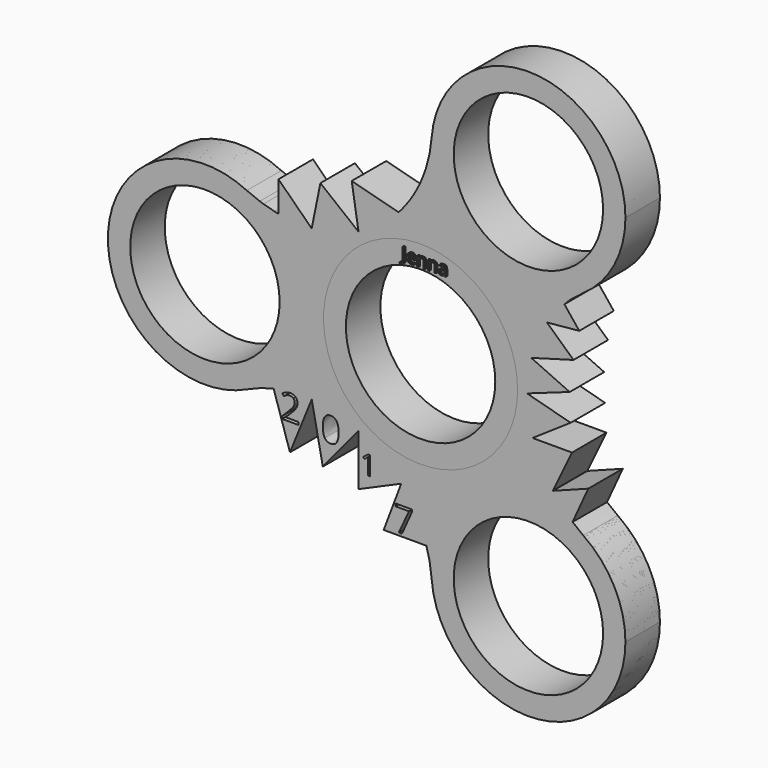
from build123d import *

# Parameters (mm, degrees)
F0_R         = 14.2875
F0_R_2       = 10.9982
F3_DEPTH     = 6.35
F1_R         = 10.9982
F1_R_2       = 14.2875
F2_TEXT_SIZE = 2.6101414632
F4_DEPTH     = 6.604


# Not quite as in the source:
# - Text() gives the source's letters only with a copy of the font that has no kerning and outlines rounded to 1/6400 em; it was checked with that copy


with BuildPart() as f3:
    # F0 (on Front) → F3 (new body)
    with BuildSketch(Plane.XZ):
        with BuildLine():
            ThreePointArc((-25.5840395423, 12.8885060377), (-19.6622207108, 7.6169710585), (-17.4625, 0))
            ThreePointArc((-17.4625, 0), (-19.6622207439, -7.616971111), (-25.5840396543, -12.8885060913))
            ThreePointArc((-25.5840396543, -12.8885060913), (-7.837759128, -13.5753968045), (1.630246118, -28.6006810957))
            ThreePointArc((1.630246118, -28.6006810957), (8.7312501488, -15.1229685276), (23.9537936189, -15.7121752949))
            ThreePointArc((23.9537936189, -15.7121752949), (15.6755180632, -1.024e-07), (23.95379345, 15.7121751791))
            ThreePointArc((23.95379345, 15.7121751791), (8.7312498422, 15.1229687047), (1.630246157, 28.6006815976))
            ThreePointArc((1.630246157, 28.6006815976), (-7.8377588563, 13.5753969614), (-25.5840395423, 12.8885060377))
        make_face()
        Circle(F0_R, mode=Mode.SUBTRACT)
        with BuildLine():
            ThreePointArc((-25.5840396543, -12.8885060913), (-19.6622207439, -7.616971111), (-17.4625, 0))
            ThreePointArc((-17.4625, 0), (-19.6622207108, 7.6169710585), (-25.5840395423, 12.8885060377))
            ThreePointArc((-25.5840395423, 12.8885060377), (-46.0375, 6.21e-08), (-25.5840396543, -12.8885060913))
        make_face()
        with Locations((-31.75, 0)):
            Circle(F0_R_2, mode=Mode.SUBTRACT)
        Circle(F0_R)
        Circle(F0_R_2, mode=Mode.SUBTRACT)
        with BuildLine():
            ThreePointArc((30.1625, 27.4963065702), (16.4276009942, 41.7731160313), (1.630246157, 28.6006815976))
            ThreePointArc((1.630246157, 28.6006815976), (8.7312498422, 15.1229687047), (23.95379345, 15.7121751791))
            ThreePointArc((23.95379345, 15.7121751791), (28.5153800905, 20.8364681775), (30.1625, 27.4963065702))
        make_face()
        with Locations((15.875, 27.4963065702)):
            Circle(F0_R_2, mode=Mode.SUBTRACT)
        with BuildLine():
            ThreePointArc((23.9537936189, -15.7121752949), (8.7312501488, -15.1229685276), (1.630246118, -28.6006810957))
            ThreePointArc((1.630246118, -28.6006810957), (16.4276007427, -41.7731160411), (30.1625, -27.4963065702))
            ThreePointArc((30.1625, -27.4963065702), (28.5153801383, -20.8364682681), (23.9537936189, -15.7121752949))
        make_face()
        with Locations((15.875, -27.4963065702)):
            Circle(F0_R_2, mode=Mode.SUBTRACT)
    extrude(amount=F3_DEPTH)

    # F2 (on face) → F4 (join)
    with BuildSketch(Plane.XZ):
        with Locations((-2.6774271391, 11.3784307614)):
            Text('Jenna', F2_TEXT_SIZE, font='Open Sans', text_align=(TextAlign.LEFT, TextAlign.BOTTOM))
    extrude(amount=F4_DEPTH)


with BuildPart() as f3b:
    # F1 (on face) → F3, piece 2 (new body)
    with BuildSketch(Plane.XZ):
        with BuildLine():
            ThreePointArc((1.6302461293, -28.6006812411), (16.4276008155, -41.7731160383), (30.1625, -27.4963065702))
            ThreePointArc((30.1625, -27.4963065702), (28.5153800921, -20.8364681805), (23.9537934556, -15.7121751829))
            ThreePointArc((23.9537934556, -15.7121751829), (8.73125, -15.1229686136), (1.6302461293, -28.6006812411))
        make_face()
        with Locations((15.875, -27.4963065702)):
            Circle(F1_R, mode=Mode.SUBTRACT)
        with BuildLine():
            ThreePointArc((1.6302461293, -28.6006812411), (8.73125, -15.1229686136), (23.9537934556, -15.7121751829))
            ThreePointArc((23.9537934556, -15.7121751829), (23.1461983486, -15.126858727), (22.3703450113, -14.5000758225))
            ThreePointArc((22.3703450113, -14.5000758225), (20.8277143031, -13.0289504814), (19.4590986494, -11.3946890384))
            ThreePointArc((19.4590986494, -11.3946890384), (17.7185481854, -8.5828594055), (16.4904950244, -5.5123892076))
            ThreePointArc((16.4904950244, -5.5123892076), (15.8803636609, -2.7861542592), (15.6755180632, 0))
            ThreePointArc((15.6755180632, 0), (15.8305224894, 2.4252097364), (16.2930133142, 4.8109529906))
            ThreePointArc((16.2930133142, 4.8109529906), (17.2447328672, 7.5713043086), (18.6071112176, 10.1537904627))
            ThreePointArc((18.6071112176, 10.1537904627), (19.7971807554, 11.8341558729), (21.1616623158, 13.3762594646))
            ThreePointArc((21.1616623158, 13.3762594646), (22.5018016331, 14.6110662389), (23.9537934556, 15.7121751829))
            ThreePointArc((23.9537934556, 15.7121751829), (8.7312498543, 15.1229686977), (1.6302461553, 28.6006815765))
            ThreePointArc((1.6302461553, 28.6006815765), (0.1447682107, 22.5639205285), (-3.2052619846, 17.3268959567))
            ThreePointArc((-3.2052619846, 17.3268959567), (-5.9528221166, 14.818154103), (-9.1356129248, 12.8913134143))
            ThreePointArc((-9.1356129248, 12.8913134143), (-12.4975441494, 11.654923986), (-16.0314960729, 11.069753771))
            ThreePointArc((-16.0314960729, 11.069753771), (-18.4857916979, 11.0563120371), (-20.921446323, 11.3585275925))
            ThreePointArc((-20.921446323, 11.3585275925), (-23.302213479, 11.9727559214), (-25.584039585, 12.8885060581))
            ThreePointArc((-25.584039585, 12.8885060581), (-19.6622207234, 7.6169710785), (-17.4625, 0))
            ThreePointArc((-17.4625, 0), (-19.6622207234, -7.6169710785), (-25.584039585, -12.8885060581))
            ThreePointArc((-25.584039585, -12.8885060581), (-23.6486295526, -12.0901240045), (-21.6372972258, -11.508945746))
            ThreePointArc((-21.6372972258, -11.508945746), (-18.8452797946, -11.08095523), (-16.0206686307, -11.0705153746))
            ThreePointArc((-16.0206686307, -11.0705153746), (-12.4954406186, -11.6554797659), (-9.1414784782, -12.8885060581))
            ThreePointArc((-9.1414784782, -12.8885060581), (-5.7422647695, -14.9779294594), (-2.8528361021, -17.7295736885))
            ThreePointArc((-2.8528361021, -17.7295736885), (-0.6379138825, -20.9527611441), (0.8721262833, -24.5603360236))
            ThreePointArc((0.8721262833, -24.5603360236), (1.3604900104, -26.5599991514), (1.6302461293, -28.6006812411))
        make_face()
        Circle(F1_R_2, mode=Mode.SUBTRACT)
        with BuildLine():
            ThreePointArc((19.4590986494, -11.3946890384), (20.8277143031, -13.0289504814), (22.3703450113, -14.5000758225))
            Line((22.3703450113, -14.5000758225), (24.6910881251, -9.410279803))
            Line((24.6910881251, -9.410279803), (19.4590986494, -11.3946890384))
        make_face()
        with BuildLine():
            Line((-5.4336530156, -24.5603360236), (0.8721262833, -24.5603360236))
            ThreePointArc((0.8721262833, -24.5603360236), (-0.6379138825, -20.9527611441), (-2.8528361021, -17.7295736885))
            Line((-2.8528361021, -17.7295736885), (-5.4336530156, -24.5603360236))
        make_face()
        Polygon((-2.7451116706, -24.1751358706), (-3.2010593322, -24.1751358706), (-1.7000003351, -20.9311673776), (-3.6744519478, -20.9311673776), (-3.6744519478, -20.5521361042), (-1.2638764849, -20.5521361042), (-1.2638764849, -20.8820043254), align=None, mode=Mode.SUBTRACT)
        with BuildLine():
            ThreePointArc((16.4904950244, -5.5123892076), (17.7185481854, -8.5828594055), (19.4590986494, -11.3946890384))
            Line((19.4590986494, -11.3946890384), (22.2941269501, -5.5123892076))
            Line((22.2941269501, -5.5123892076), (16.4904950244, -5.5123892076))
        make_face()
        with BuildLine():
            Line((-9.1414784782, -20.4766951501), (-2.8528361021, -17.7295736885))
            ThreePointArc((-2.8528361021, -17.7295736885), (-5.7422647695, -14.9779294594), (-9.1414784782, -12.8885060581))
            Line((-9.1414784782, -12.8885060581), (-9.1414784782, -20.4766951501))
        make_face()
        with BuildLine():
            Line((-7.4396296546, -15.5139071946), (-7.4396296546, -18.2712860405))
            Line((-7.4396296546, -18.2712860405), (-7.7449992532, -18.2712860405))
            Line((-7.7449992532, -18.2712860405), (-7.7449992532, -16.3062990582))
            add(Edge.make_bspline(
                [(-7.7449992532, -16.3062990582), (-7.7449992532, -16.0606756854), (-7.7299118224, -15.8422096879)],
                knots=[0, 0, 0, 1, 1, 1], degree=2))
            add(Edge.make_bspline(
                [(-7.7299118224, -15.8422096879), (-7.7691391424, -15.8820405052), (-7.8183241667, -15.9251905571)],
                knots=[0, 0, 0, 1, 1, 1], degree=2))
            add(Edge.make_bspline(
                [(-7.8183241667, -15.9251905571), (-7.867509191, -15.9683406091), (-8.2670243575, -16.2930221191)],
                knots=[0, 0, 0, 1, 1, 1], degree=2))
            Line((-8.2670243575, -16.2930221191), (-8.4329860959, -16.0781771051))
            Line((-8.4329860959, -16.0781771051), (-7.7033579443, -15.5139071946))
            Line((-7.7033579443, -15.5139071946), (-7.4396296546, -15.5139071946))
        make_face(mode=Mode.SUBTRACT)
        with BuildLine():
            ThreePointArc((15.6755180632, 0), (15.8803636609, -2.7861542592), (16.4904950244, -5.5123892076))
            Line((16.4904950244, -5.5123892076), (22.0935102552, -1.7202883027))
            Line((22.0935102552, -1.7202883027), (15.6755180632, 0))
        make_face()
        with BuildLine():
            Line((-14.3941845745, -19.2679259926), (-9.1414784782, -12.8885060581))
            ThreePointArc((-9.1414784782, -12.8885060581), (-12.4954406186, -11.6554797659), (-16.0206686307, -11.0705153746))
            Line((-16.0206686307, -11.0705153746), (-14.3941845745, -19.2679259926))
        make_face()
        with BuildLine():
            add(Edge.make_bspline(
                [(-12.3585854696, -12.7484392756), (-12.0600410802, -13.2152049207), (-12.0600410802, -14.099236623)],
                knots=[0, 0, 0, 1, 1, 1], degree=2))
            add(Edge.make_bspline(
                [(-12.0600410802, -14.099236623), (-12.0600410802, -15.0157524299), (-12.3489175813, -15.4678228848)],
                knots=[0, 0, 0, 1, 1, 1], degree=2))
            add(Edge.make_bspline(
                [(-12.3489175813, -15.4678228848), (-12.6377940825, -15.9198933397), (-13.2325625681, -15.9198933397)],
                knots=[0, 0, 0, 1, 1, 1], degree=2))
            add(Edge.make_bspline(
                [(-13.2325625681, -15.9198933397), (-13.8025812598, -15.9198933397), (-14.0999655026, -15.45699485)],
                knots=[0, 0, 0, 1, 1, 1], degree=2))
            add(Edge.make_bspline(
                [(-14.0999655026, -15.45699485), (-14.3973497454, -14.9940963602), (-14.3973497454, -14.099236623)],
                knots=[0, 0, 0, 1, 1, 1], degree=2))
            add(Edge.make_bspline(
                [(-14.3973497454, -14.099236623), (-14.3973497454, -13.1765333677), (-14.1096333908, -12.7291034991)],
                knots=[0, 0, 0, 1, 1, 1], degree=2))
            add(Edge.make_bspline(
                [(-14.1096333908, -12.7291034991), (-13.8219170363, -12.2816736305), (-13.2325625681, -12.2816736305)],
                knots=[0, 0, 0, 1, 1, 1], degree=2))
            add(Edge.make_bspline(
                [(-13.2325625681, -12.2816736305), (-12.657129859, -12.2816736305), (-12.3585854696, -12.7484392756)],
                knots=[0, 0, 0, 1, 1, 1], degree=2))
        make_face(mode=Mode.SUBTRACT)
        with BuildLine():
            ThreePointArc((16.2930133142, 4.8109529906), (15.8305224894, 2.4252097364), (15.6755180632, 0))
            Line((15.6755180632, 0), (21.9561289996, 2.2296286188))
            Line((21.9561289996, 2.2296286188), (16.2930133142, 4.8109529906))
        make_face()
        with BuildLine():
            Line((-19.2302669593, -18.9881071762), (-16.0206686307, -11.0705153746))
            ThreePointArc((-16.0206686307, -11.0705153746), (-18.8452797946, -11.08095523), (-21.6372972258, -11.508945746))
            Line((-21.6372972258, -11.508945746), (-19.2302669593, -18.9881071762))
        make_face()
        with BuildLine():
            Line((-17.9606955723, -14.6407701649), (-17.9606955723, -15.0293112754))
            Line((-17.9606955723, -15.0293112754), (-20.3864522355, -15.0293112754))
            Line((-20.3864522355, -15.0293112754), (-20.3864522355, -14.6682346093))
            Line((-20.3864522355, -14.6682346093), (-19.4146955702, -13.6916312774))
            add(Edge.make_bspline(
                [(-19.4146955702, -13.6916312774), (-18.9704177931, -13.2416990558), (-18.8290566822, -13.0498518338)],
                knots=[0, 0, 0, 1, 1, 1], degree=2))
            add(Edge.make_bspline(
                [(-18.8290566822, -13.0498518338), (-18.6876955712, -12.8580046119), (-18.6170150158, -12.6762546122)],
                knots=[0, 0, 0, 1, 1, 1], degree=2))
            add(Edge.make_bspline(
                [(-18.6170150158, -12.6762546122), (-18.5463344603, -12.4945046124), (-18.5463344603, -12.2852901683)],
                knots=[0, 0, 0, 1, 1, 1], degree=2))
            add(Edge.make_bspline(
                [(-18.5463344603, -12.2852901683), (-18.5463344603, -11.989643502), (-18.7256611267, -11.8167790578)],
                knots=[0, 0, 0, 1, 1, 1], degree=2))
            add(Edge.make_bspline(
                [(-18.7256611267, -11.8167790578), (-18.9049877932, -11.6439146136), (-19.2232522371, -11.6439146136)],
                knots=[0, 0, 0, 1, 1, 1], degree=2))
            add(Edge.make_bspline(
                [(-19.2232522371, -11.6439146136), (-19.4526611257, -11.6439146136), (-19.6586444587, -11.7198457246)],
                knots=[0, 0, 0, 1, 1, 1], degree=2))
            add(Edge.make_bspline(
                [(-19.6586444587, -11.7198457246), (-19.8646277918, -11.7957768357), (-20.1166544581, -11.9952979465)],
                knots=[0, 0, 0, 1, 1, 1], degree=2))
            Line((-20.1166544581, -11.9952979465), (-20.3387933466, -11.7101523913))
            add(Edge.make_bspline(
                [(-20.3387933466, -11.7101523913), (-19.8290855696, -11.2860690586), (-19.2280989038, -11.2860690586)],
                knots=[0, 0, 0, 1, 1, 1], degree=2))
            add(Edge.make_bspline(
                [(-19.2280989038, -11.2860690586), (-18.7078900157, -11.2860690586), (-18.4126472383, -11.552231836)],
                knots=[0, 0, 0, 1, 1, 1], degree=2))
            add(Edge.make_bspline(
                [(-18.4126472383, -11.552231836), (-18.117404461, -11.8183946134), (-18.117404461, -12.2675190572)],
                knots=[0, 0, 0, 1, 1, 1], degree=2))
            add(Edge.make_bspline(
                [(-18.117404461, -12.2675190572), (-18.117404461, -12.61890239), (-18.3145022385, -12.9622079451)],
                knots=[0, 0, 0, 1, 1, 1], degree=2))
            add(Edge.make_bspline(
                [(-18.3145022385, -12.9622079451), (-18.5116000159, -13.3055135001), (-19.0511955707, -13.8305690549)],
                knots=[0, 0, 0, 1, 1, 1], degree=2))
            Line((-19.0511955707, -13.8305690549), (-19.8589733473, -14.6205757205))
            Line((-19.8589733473, -14.6205757205), (-19.8589733473, -14.6407701649))
            Line((-19.8589733473, -14.6407701649), (-17.9606955723, -14.6407701649))
        make_face(mode=Mode.SUBTRACT)
        with BuildLine():
            ThreePointArc((18.6071112176, 10.1537904627), (17.2447328672, 7.5713043086), (16.2930133142, 4.8109529906))
            Line((16.2930133142, 4.8109529906), (22.5192476064, 6.5634795465))
            Line((22.5192476064, 6.5634795465), (18.6071112176, 10.1537904627))
        make_face()
        with BuildLine():
            ThreePointArc((21.1616623158, 13.3762594646), (19.7971807554, 11.8341558729), (18.6071112176, 10.1537904627))
            Line((18.6071112176, 10.1537904627), (23.3653895557, 10.6105785817))
            Line((23.3653895557, 10.6105785817), (21.1616623158, 13.3762594646))
        make_face()
        with BuildLine():
            ThreePointArc((-25.584039585, 12.8885060581), (-46.0375, 0), (-25.584039585, -12.8885060581))
            ThreePointArc((-25.584039585, -12.8885060581), (-19.6622207234, -7.6169710785), (-17.4625, 0))
            ThreePointArc((-17.4625, 0), (-19.6622207234, 7.6169710785), (-25.584039585, 12.8885060581))
        make_face()
        with Locations((-31.75, 0)):
            Circle(F1_R, mode=Mode.SUBTRACT)
        with BuildLine():
            ThreePointArc((1.6302461553, 28.6006815765), (8.7312498543, 15.1229686977), (23.9537934556, 15.7121751829))
            ThreePointArc((23.9537934556, 15.7121751829), (28.5153800921, 20.8364681805), (30.1625, 27.4963065702))
            ThreePointArc((30.1625, 27.4963065702), (16.4276009836, 41.7731160318), (1.6302461553, 28.6006815765))
        make_face()
        with Locations((15.875, 27.4963065702)):
            Circle(F1_R, mode=Mode.SUBTRACT)
        with BuildLine():
            Line((-20.921446323, 15.861414403), (-20.921446323, 11.3585275925))
            ThreePointArc((-20.921446323, 11.3585275925), (-18.4857916979, 11.0563120371), (-16.0314960729, 11.069753771))
            Line((-16.0314960729, 11.069753771), (-20.921446323, 15.861414403))
        make_face()
        with BuildLine():
            Line((-14.7465616465, 17.369935289), (-16.0314960729, 11.069753771))
            ThreePointArc((-16.0314960729, 11.069753771), (-12.4975441494, 11.654923986), (-9.1356129248, 12.8913134143))
            Line((-9.1356129248, 12.8913134143), (-14.7465616465, 17.369935289))
        make_face()
        with BuildLine():
            ThreePointArc((-9.1356129248, 12.8913134143), (-5.9528221166, 14.818154103), (-3.2052619846, 17.3268959567))
            Line((-3.2052619846, 17.3268959567), (-10.1375561208, 19.1490314901))
            Line((-10.1375561208, 19.1490314901), (-9.1356129248, 12.8913134143))
        make_face()
    extrude(amount=F3_DEPTH)


solid = Compound([f3.part, f3b.part])
